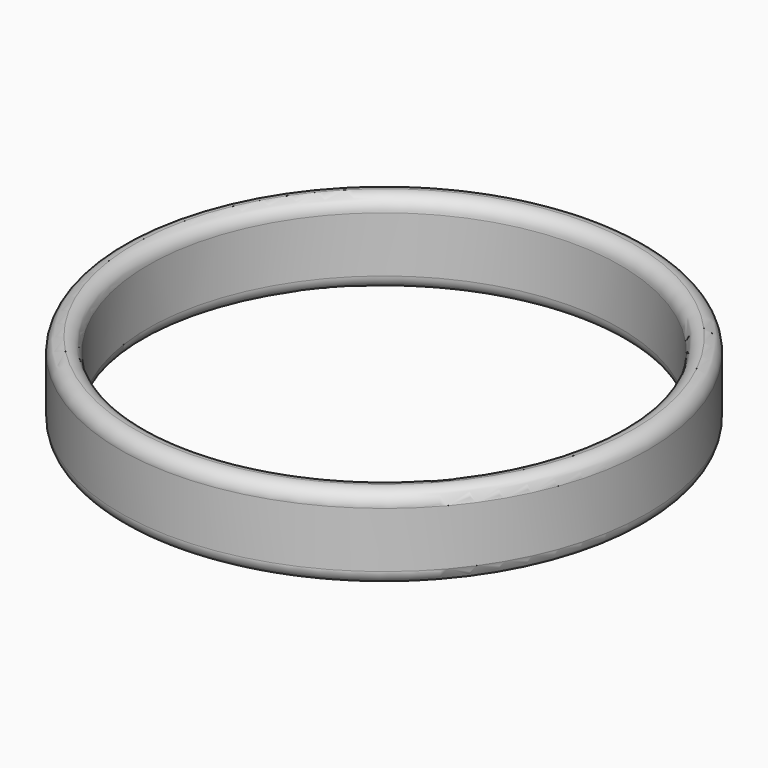
from build123d import *

# Parameters (mm, degrees)
F0_R     = 9.5
F0_R_2   = 8.5
F1_DEPTH = 3
F2_R     = 0.49999


# Not quite as in the source:
# - a fillet or chamfer is up to 0.001 mm smaller than in the source, because OpenCascade refuses the exact size


with BuildPart() as f1:
    # F0 (on Top) → F1 (new body)
    with BuildSketch(Plane.XY):
        Circle(F0_R)
        Circle(F0_R_2, mode=Mode.SUBTRACT)
    extrude(amount=F1_DEPTH)

    # F2 (radius 0.5 in the source; OpenCascade refuses exactly that, so slightly less here)
    f2_edges = [f1.edges().sort_by_distance(p)[0] for p in [
        (-9.5, 0, 3),
        (-8.5, 0, 3),
        (-9.5, 0, 0),
        (-8.5, 0, 0),
    ]]
    fillet(f2_edges, radius=F2_R)


solid = f1.part
